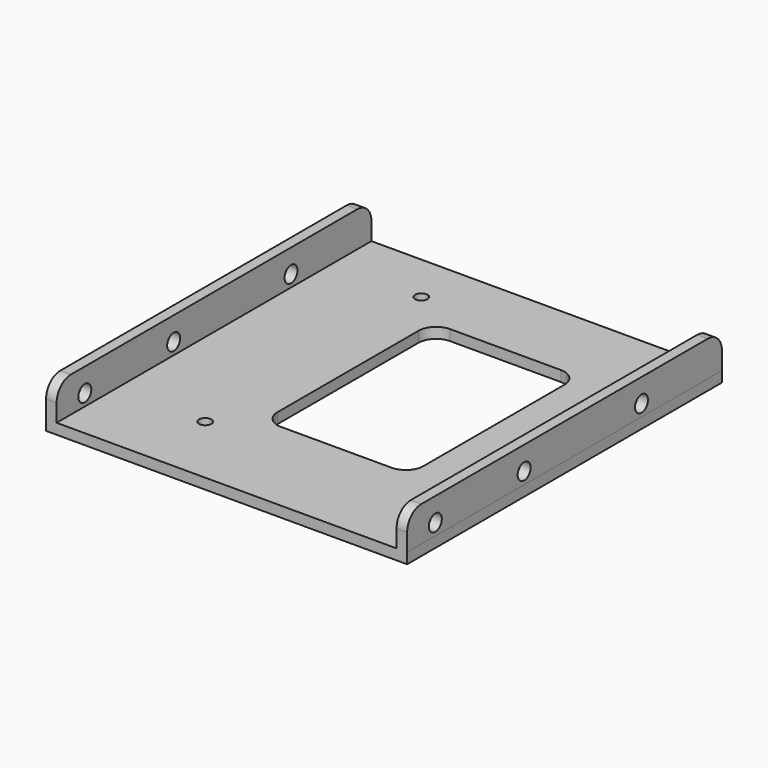
from build123d import *

# Parameters (mm, degrees)
F0_W      = 102.4
F0_H      = 147
F1_DEPTH  = 3
F2_W      = 3
F2_H      = 147
F3_DEPTH  = 10
F5_R      = 2.3
F6_DEPTH  = 102.401
F7_R      = 1.75
F8_DEPTH  = 3.001
F9_W      = 41.4
F9_H      = 60
F9_W_2    = 96.3999993775
F9_H_2    = 35.4163302109
F10_DEPTH = 12.5
F11_R     = 5


# Not quite as in the source:
# - a pattern or mirror of a feature is missing from the dataset's text; its kind, count and spacing are read off the source's solid
# - a feature names something its author has since deleted; it is built from what else it names


with BuildPart() as f1:
    # F0 (on Top) → F1 (new body)
    with BuildSketch(Plane.XY):
        with Locations((-12.3022546887, 26.2855888009)):
            Rectangle(F0_W, F0_H)
    extrude(amount=F1_DEPTH)

    # F2 (on face) → F3 (join)
    with BuildSketch(Plane.XY.offset(3)):
        with Locations((-62.0022546887, 26.2855888009)):
            Rectangle(F2_W, F2_H)
    f3 = extrude(amount=F3_DEPTH)

    # F3_copies: F3 across plane
    add(f3.mirror(Plane(origin=(-12.302255, 0, 0), x_dir=(0, 0, 1), z_dir=(1, 0, 0))))

    # F5 (on face) → F6 (cut, through all)
    with BuildSketch(Plane(origin=(-63.5022546887, 0, 0), x_dir=(0, -1, 0), z_dir=(-1, 0, 0))):
        with Locations((1.8144111991, 6.35)):
            Circle(F5_R)
        with Locations((-29.6755888009, 6.35)):
            Circle(F5_R)
        with Locations((-71.2855888009, 6.35)):
            Circle(F5_R)
    extrude(amount=-F6_DEPTH, mode=Mode.SUBTRACT)

    # F7 (on face) → F8 (cut, through all)
    with BuildSketch(Plane.XY.offset(3)):
        with Locations((26.5577453113, 9.1855888009)):
            Circle(F7_R)
        with Locations((-35.1622546887, 9.1855888009)):
            Circle(F7_R)
        with Locations((-35.1622546887, 85.7855888009)):
            Circle(F7_R)
        with Locations((26.5577453113, 85.7855888009)):
            Circle(F7_R)
    extrude(amount=-F8_DEPTH, mode=Mode.SUBTRACT)

    # F9 (on face) → F10 (cut, symmetric)
    with BuildSketch(Plane.XY.offset(3)):
        with Locations((-4.8022546887, 47.7176743746)):
            Rectangle(F9_W, F9_H)
        with Locations((-12.302255, -29.5062460937)):
            Rectangle(F9_W_2, F9_H_2)
        Polygon((-71.4376792312, -51.2489080429), (43.8891761005, -51.2489080429), (43.8891761005, -11.7980809882), (35.8977446887, -11.7980809882), (35.8977446887, -47.2144111991), (-60.5022546887, -47.2144111991), (-60.5022546887, -11.7980809882), (-71.4376792312, -11.7980809882), align=None)
    extrude(amount=F10_DEPTH, both=True, mode=Mode.SUBTRACT)

    # F11
    f11_edges = [f1.edges().sort_by_distance(p)[0] for p in [
        (-62.002255, 99.785589, 13),
        (-62.002255, -11.798081, 13),
        (15.897745, 17.717674, 1.5),
        (-25.502255, 17.717674, 1.5),
        (-25.502255, 77.717674, 1.5),
        (15.897745, 77.717674, 1.5),
        (37.397745, 99.785589, 13),
        (37.397745, -11.798081, 13),
    ]]
    fillet(f11_edges, radius=F11_R)


solid = f1.part
